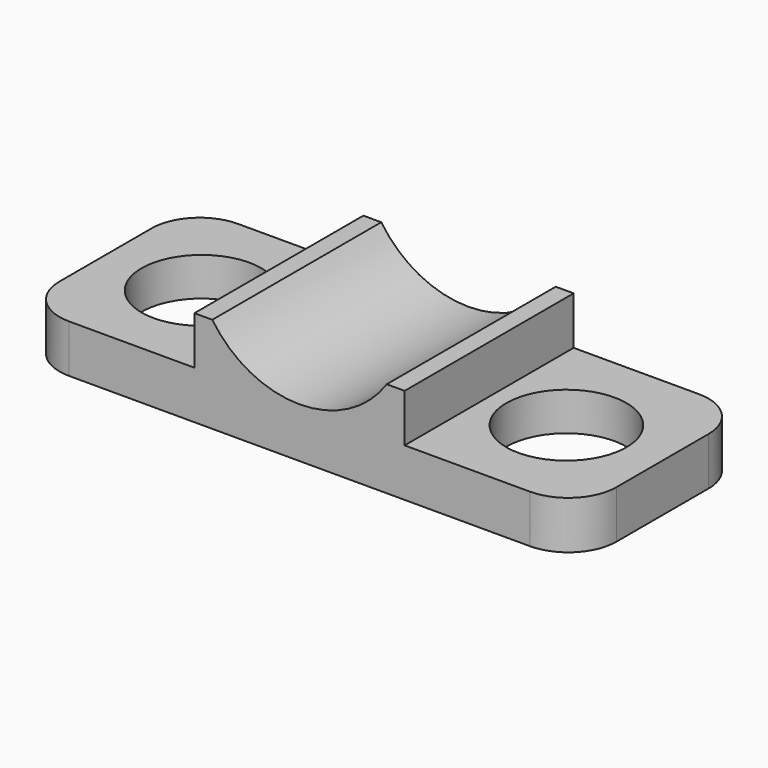
from build123d import *

# Parameters (mm, degrees)
F2_DEPTH = 11
F3_R     = 6.25
F4_DEPTH = 5.001
F5_R     = 5
F6_R     = 8.6
F7_DEPTH = 1


# Not quite as in the source:
# - a pattern or mirror of a feature is missing from the dataset's text; its kind, count and spacing are read off the source's solid


with BuildPart() as f2:
    # F1 (on Front) → F2 (new body, symmetric)
    with BuildSketch(Plane.XZ):
        with BuildLine():
            ThreePointArc((9.0862533533, 5), (0, 0.2), (-9.0862533533, 5))
            Line((-9.0862533533, 5), (-10.95, 5))
            Line((-10.95, 5), (-10.95, 0))
            Line((-10.95, 0), (-29, 0))
            Line((-29, 0), (-29, -5))
            Line((-29, -5), (29, -5))
            Line((29, -5), (29, 0))
            Line((29, 0), (10.95, 0))
            Line((10.95, 0), (10.95, 5))
            Line((10.95, 5), (9.0862533533, 5))
        make_face()
    extrude(amount=F2_DEPTH, both=True)

    # F3 (on Top) → F4 (cut, through all)
    with BuildSketch(Plane.XY):
        with Locations((-19, 0)):
            Circle(F3_R)
    f4 = extrude(amount=-F4_DEPTH, mode=Mode.SUBTRACT)

    # F4_copies: F4 across plane
    add(f4.mirror(Plane(origin=(0, 0, 0), x_dir=(0, 0, 1), z_dir=(1, 0, 0))), mode=Mode.SUBTRACT)

    # F5
    f5_edges = [f2.edges().sort_by_distance(p)[0] for p in [
        (-29, -11, -2.5),
        (-29, 11, -2.5),
        (29, -11, -2.5),
        (29, 11, -2.5),
    ]]
    fillet(f5_edges, radius=F5_R)

    # F6 (on face) → F7 (cut)
    with BuildSketch(Plane(origin=(0, 0, -5), x_dir=(1, 0, 0), z_dir=(0, 0, -1))):
        with Locations((-19, 0)):
            Circle(F6_R)
        with Locations((19, 0)):
            Circle(F6_R)
    extrude(amount=-F7_DEPTH, mode=Mode.SUBTRACT)


solid = f2.part
